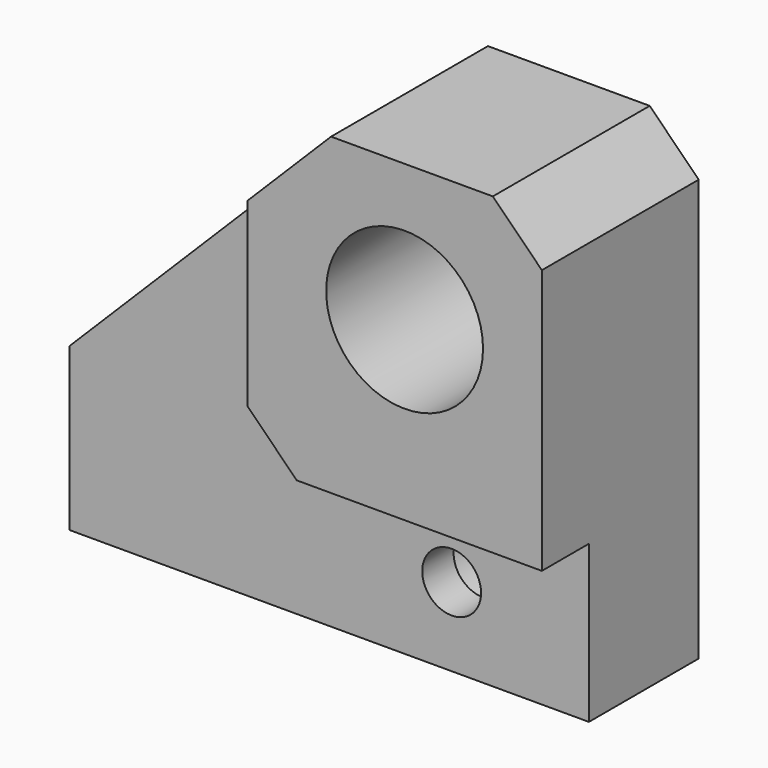
from build123d import *

# Parameters (mm, degrees)
F0_W      = 168.275
F0_H      = 152.4
F1_DEPTH  = 44.45
F3_DEPTH  = 44.451
F4_W      = 23.8125
F4_H      = 19.05
F5_DEPTH  = 152.401
F7_DEPTH  = 19.05
F8_R      = 25.4
F9_DEPTH  = 63.501
F10_R     = 9.525
F11_DEPTH = 44.451
F12_R     = 15.875
F12_R_2   = 9.525
F13_DEPTH = 31.75


with BuildPart() as f1:
    # F0 (on Front) → F1 (new body)
    with BuildSketch(Plane.XZ):
        with Locations((-5.8413036168, -23.7527878196)):
            Rectangle(F0_W, F0_H)
    extrude(amount=F1_DEPTH)

    # F2 (on face) → F3 (cut, through all)
    with BuildSketch(Plane.XZ.offset(44.45)):
        Polygon((-89.9788036168, 52.4472121804), (-89.9788036168, -47.5652878196), (10.0336963832, 52.4472121804), align=None)
    extrude(amount=-F3_DEPTH, mode=Mode.SUBTRACT)

    # F4 (on face) → F5 (cut, through all)
    with BuildSketch(Plane(origin=(0, 0, -99.9527878196), x_dir=(1, 0, 0), z_dir=(0, 0, -1))):
        with Locations((-49.4975536168, 9.525)):
            Rectangle(F4_W, F4_H)
    extrude(amount=-F5_DEPTH, mode=Mode.SUBTRACT)

    # F6 (on face) → F7 (join)
    with BuildSketch(Plane.XZ.offset(44.45)):
        Polygon((-1.0788036168, -49.1527878196), (78.2961963832, -49.1527878196), (78.2961963832, 52.4472121804), (10.0336963832, 52.4472121804), (-16.9538036168, 25.4597121804), (-16.9538036168, -33.2777878196), align=None)
    extrude(amount=F7_DEPTH)

    # F8 (on face) → F9 (cut, through all)
    with BuildSketch(Plane.XZ.offset(63.5)):
        with Locations((33.8461963832, 7.9972121804)):
            Circle(F8_R)
        Polygon((78.2961963832, 52.4472121804), (62.4211963832, 52.4472121804), (78.2961963832, 36.5722121804), align=None)
    extrude(amount=-F9_DEPTH, mode=Mode.SUBTRACT)

    # F10 (on face) → F11 (cut, through all)
    with BuildSketch(Plane.XZ.offset(44.45)):
        with Locations((33.8461963832, -74.5527878196)):
            Circle(F10_R)
    extrude(amount=-F11_DEPTH, mode=Mode.SUBTRACT)

    # F12 (on face) → F13 (cut)
    with BuildSketch(Plane(origin=(0, 0, 0), x_dir=(-1, 0, 0), z_dir=(0, 1, 0))):
        with Locations((-33.8461963832, -74.5527878196)):
            Circle(F12_R)
        with Locations((-33.8461963832, -74.5527878196)):
            Circle(F12_R_2, mode=Mode.SUBTRACT)
    extrude(amount=-F13_DEPTH, mode=Mode.SUBTRACT)


solid = f1.part
